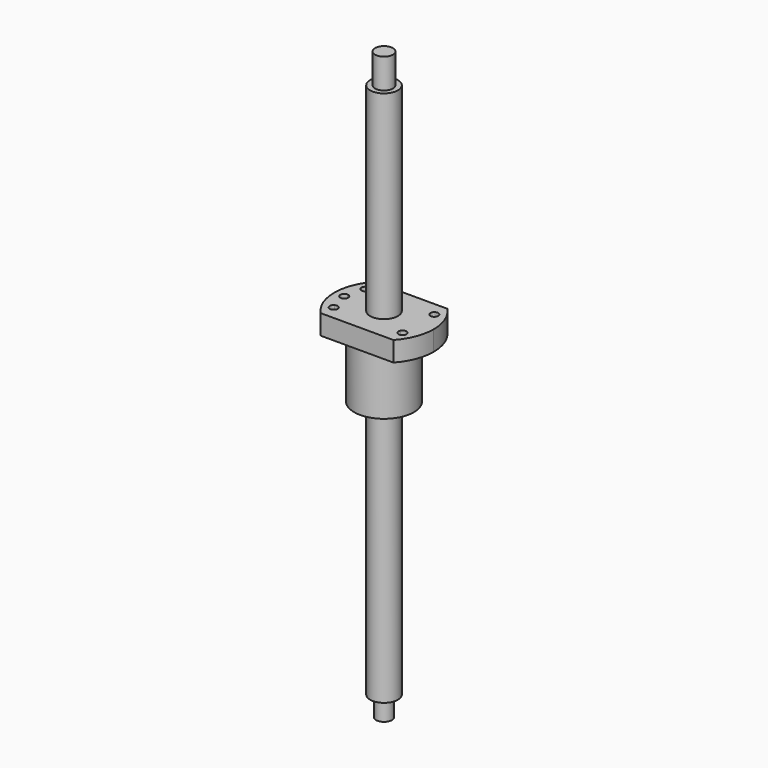
from build123d import *

# Parameters (mm, degrees)
F0_R          = 15
F1_DEPTH      = 30
F2_R          = 15
F3_DEPTH      = 10
F4_DEPTH      = 25
F6_R          = 7
F7_DEPTH      = 130
F7_DEPTH_BACK = 140
F8_R          = 4
F9_DEPTH      = 10
F10_R         = 4.5
F11_DEPTH     = 15


# Not quite as in the source:
# - a pattern or mirror of a feature is missing from the dataset's text; its kind, count and spacing are read off the source's solid


with BuildPart() as f1:
    # F0 (on Top) → F1 (new body)
    with BuildSketch(Plane.XY):
        Circle(F0_R)
    extrude(amount=F1_DEPTH)

    # F2 (on face) → F3 (join)
    with BuildSketch(Plane.XY.offset(30)):
        with BuildLine():
            ThreePointArc((10.5356537529, -17), (17.4744538549, -9.7284871625), (20, 0))
            ThreePointArc((20, 0), (17.4744538549, 9.7284871625), (10.5356537529, 17))
            Line((10.5356537529, 17), (-10.5356537529, 17))
            ThreePointArc((-10.5356537529, 17), (-16.9661727605, 10.5900416364), (-19.9, 1.9974984355))
            ThreePointArc((-19.9, 1.9974984355), (-18.5508623254, 1.3784048752), (-18, 0))
            ThreePointArc((-18, 0), (-18.5508623254, -1.3784048752), (-19.9, -1.9974984355))
            ThreePointArc((-19.9, -1.9974984355), (-16.9661727605, -10.5900416364), (-10.5356537529, -17))
            Line((-10.5356537529, -17), (10.5356537529, -17))
        make_face()
        Circle(F2_R, mode=Mode.SUBTRACT)
        with BuildLine():
            ThreePointArc((10.5356537529, 17), (17.4744538549, 9.7284871625), (20, 0))
            ThreePointArc((20, 0), (17.4744538549, -9.7284871625), (10.5356537529, -17))
            Line((10.5356537529, -17), (18.3303027798, -17))
            ThreePointArc((18.3303027798, -17), (23.2729195579, -9.1307839342), (25, 0))
            ThreePointArc((25, 0), (23.2729195579, 9.1307839342), (18.3303027798, 17))
            Line((18.3303027798, 17), (10.5356537529, 17))
        make_face()
        with BuildLine():
            ThreePointArc((-19.9, 1.9974984355), (-16.9661727605, 10.5900416364), (-10.5356537529, 17))
            Line((-10.5356537529, 17), (-18.3303027798, 17))
            ThreePointArc((-18.3303027798, 17), (-25, 0), (-18.3303027798, -17))
            Line((-18.3303027798, -17), (-10.5356537529, -17))
            ThreePointArc((-10.5356537529, -17), (-16.9661727605, -10.5900416364), (-19.9, -1.9974984355))
            ThreePointArc((-19.9, -1.9974984355), (-22, 0), (-19.9, 1.9974984355))
        make_face()
        with BuildLine():
            ThreePointArc((-18, 0), (-18.5508623254, 1.3784048752), (-19.9, 1.9974984355))
            ThreePointArc((-19.9, 1.9974984355), (-20, 0), (-19.9, -1.9974984355))
            ThreePointArc((-19.9, -1.9974984355), (-18.5508623254, -1.3784048752), (-18, 0))
        make_face()
        with BuildLine():
            ThreePointArc((-19.9, -1.9974984355), (-20, 0), (-19.9, 1.9974984355))
            ThreePointArc((-19.9, 1.9974984355), (-22, 0), (-19.9, -1.9974984355))
        make_face()
        Circle(F2_R)
    extrude(amount=F3_DEPTH)

    # F2 (on face) → F4 (cut)
    with BuildSketch(Plane.XY.offset(30)):
        with BuildLine():
            ThreePointArc((-18, 0), (-18.5508623254, 1.3784048752), (-19.9, 1.9974984355))
            ThreePointArc((-19.9, 1.9974984355), (-20, 0), (-19.9, -1.9974984355))
            ThreePointArc((-19.9, -1.9974984355), (-18.5508623254, -1.3784048752), (-18, 0))
        make_face()
        with BuildLine():
            ThreePointArc((-19.9, -1.9974984355), (-20, 0), (-19.9, 1.9974984355))
            ThreePointArc((-19.9, 1.9974984355), (-22, 0), (-19.9, -1.9974984355))
        make_face()
    f4 = extrude(amount=F4_DEPTH, mode=Mode.SUBTRACT)

    # F4_copies: F4 across plane
    add(f4.mirror(Plane(origin=(0, 0, 0), x_dir=(-0.9659258263, -0.2588190451, 0), z_dir=(0.2588190451, -0.9659258263, 0))), mode=Mode.SUBTRACT)

    # F4_copies1: F4 across plane
    add(f4.mirror(Plane(origin=(0, 0, 0), x_dir=(0.9659258263, -0.2588190451, 0), z_dir=(0.2588190451, 0.9659258263, 0))), mode=Mode.SUBTRACT)

    # F4_copies2: F4 across plane
    add(f4.mirror(Plane(origin=(0, 0, 0), x_dir=(0.2588190451, 0.9659258263, 0), z_dir=(0.9659258263, -0.2588190451, 0))), mode=Mode.SUBTRACT)

    # F4_copies3: F4 across plane
    add(f4.mirror(Plane(origin=(0, 0, 0), x_dir=(-0.2588190451, 0.9659258263, 0), z_dir=(0.9659258263, 0.2588190451, 0))), mode=Mode.SUBTRACT)

    # F6 (on face) → F7 (join, two sides)
    with BuildSketch(Plane(origin=(0, 0, 0), x_dir=(1, 0, 0), z_dir=(0, 0, -1))) as f7_sk:
        Circle(F6_R)
    extrude(amount=F7_DEPTH)
    extrude(f7_sk.sketch, amount=-F7_DEPTH_BACK)

    # F8 (on face) → F9 (join)
    with BuildSketch(Plane(origin=(0, 0, -130), x_dir=(1, 0, 0), z_dir=(0, 0, -1))):
        Circle(F8_R)
    extrude(amount=F9_DEPTH)

    # F10 (on face) → F11 (join)
    with BuildSketch(Plane.XY.offset(140)):
        Circle(F10_R)
    extrude(amount=F11_DEPTH)


solid = f1.part
